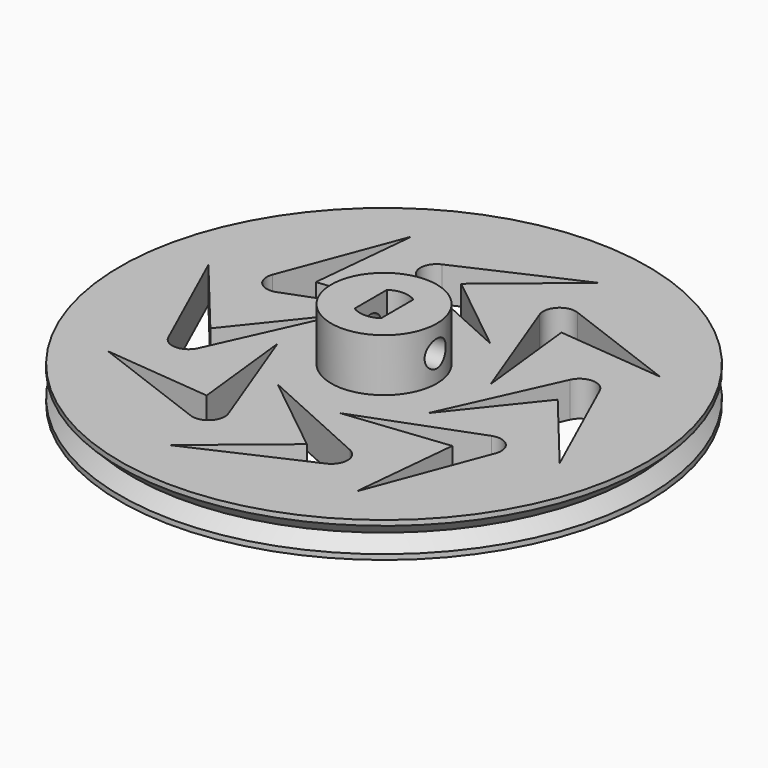
from build123d import *

# Parameters (mm, degrees)
F0_R             = 30
F0_R_2           = 6
F1_DEPTH         = 4
F2_DEPTH         = 6
F3_W             = 3
F3_H             = 4.6
F4_DEPTH         = 9.4
F8_R             = 1.5
F9_DEPTH         = 49.2
F11_DEPTH        = 4
F11_COPIES_COUNT = 8


# Not quite as in the source:
# - a pattern or mirror of a feature is missing from the dataset's text; its kind, count and spacing are read off the source's solid


with BuildPart() as f1:
    # F0 (on Top) → F1 (new body)
    with BuildSketch(Plane.XY):
        Circle(F0_R)
        Circle(F0_R_2, mode=Mode.SUBTRACT)
        Circle(F0_R_2)
    extrude(amount=-F1_DEPTH)

    # F0 (on Top) → F2 (join)
    with BuildSketch(Plane.XY):
        Circle(F0_R_2)
    extrude(amount=F2_DEPTH)

    # F3 (on face) → F4 (cut)
    with BuildSketch(Plane.XY.offset(6)):
        with BuildLine():
            Line((1.5, -2.3), (-1.5, -2.3))
            ThreePointArc((-1.5, -2.3), (0, -2.75), (1.5, -2.3))
        make_face()
        Rectangle(F3_W, F3_H)
        with BuildLine():
            ThreePointArc((1.5, 2.3), (0, 2.75), (-1.5, 2.3))
            Line((-1.5, 2.3), (1.5, 2.3))
        make_face()
    extrude(amount=-F4_DEPTH, mode=Mode.SUBTRACT)

    # F5 (on Front) → F6 (revolve, cut)
    with BuildSketch(Plane.XZ):
        Polygon((-30, -0.5857864376), (-30, -3.4142135624), (-28.5857864376, -2), align=None)
    revolve(axis=Axis((0, 0, -0.1510307193), (0, 0, -1)), mode=Mode.SUBTRACT)

    # F8 (on offset) → F9 (cut)
    with BuildSketch(Plane.YZ.offset(25)):
        with Locations((0, 3)):
            Circle(F8_R)
    extrude(amount=-F9_DEPTH, mode=Mode.SUBTRACT)

    # F10 (on face) → F11 (cut, through all)
    with BuildSketch(Plane.XY):
        with BuildLine():
            Line((-4.2793955654, 16.3180977106), (5.1502715485, 24.0833689493))
            Line((5.1502715485, 24.0833689493), (-7.9538393766, 18.1553196162))
            ThreePointArc((-7.9538393766, 18.1553196162), (-9.040407042, 16.47119876), (-7.9538393766, 14.7870779037))
            Line((-7.9538393766, 14.7870779037), (4.9067144282, 8.9692091569))
            Line((4.9067144282, 8.9692091569), (-4.2793955654, 16.3180977106))
        make_face()
    f11 = extrude(amount=-F11_DEPTH, mode=Mode.SUBTRACT)

    # F11_copies: F11 ×8 about axis
    f11_copies_axis = Axis((0, 0, 0), (0, 0, 1))
    for i in range(1, F11_COPIES_COUNT):
        add(f11.rotate(f11_copies_axis, i * 360 / F11_COPIES_COUNT), mode=Mode.SUBTRACT)


solid = f1.part
